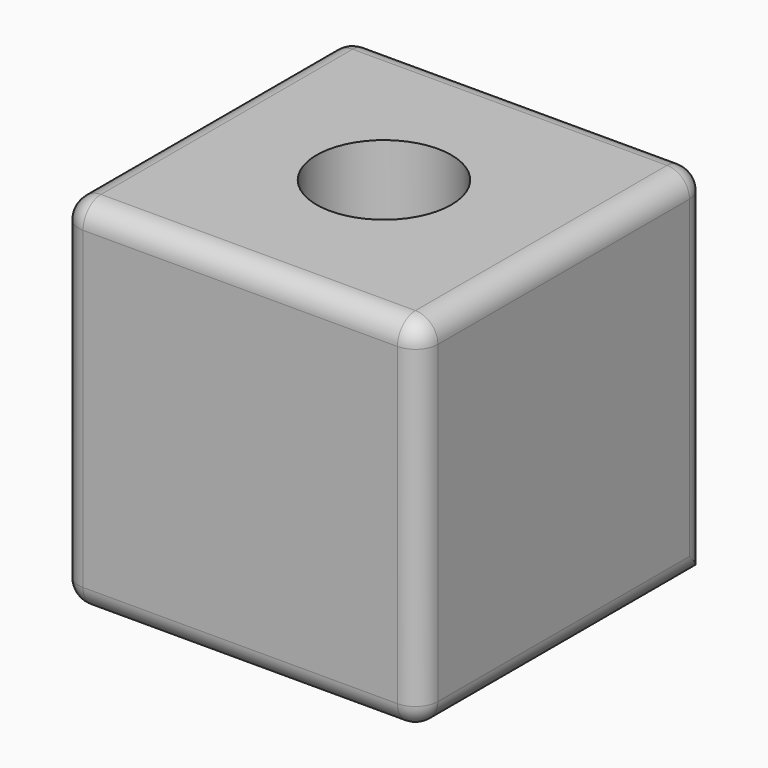
from build123d import *

# Parameters (mm, degrees)
F0_W        = 80
F0_H        = 80
F1_DEPTH    = 80
F2_R        = 5
F3_T1_DEPTH = 82.5
F3_S5_W     = 5.1
F3_S5_H     = 5.1
F3_T6_DEPTH = 5.1
F4_R        = 15
F5_DEPTH    = 80.0010001


# Not quite as in the source:
# - a fillet or chamfer that OpenCascade refuses, or shapes differently, is made with other operations: its cross-section is extruded or revolved along the edge and cut away or added


with BuildPart() as f1:
    # F0 (on Top) → F1 (new body)
    with BuildSketch(Plane.XY):
        Rectangle(F0_W, F0_H)
    extrude(amount=F1_DEPTH)

    # F2
    f2_edges = [f1.edges().sort_by_distance(p)[0] for p in [
        (0, 40, 80),
        (-40, 0, 80),
        (40, 0, 80),
        (0, -40, 80),
        (-40, 40, 40),
        (-40, 0, 0),
        (-40, -40, 40),
        (40, -40, 40),
        (0, -40, 0),
        (40, 40, 40),
        (0, 40, 0),
    ]]
    fillet(f2_edges, radius=F2_R)

    # F3: fillet of radius 5 on 8 edges, made by hand

    # F3_s2 → F3_t1 (cut)
    with BuildSketch(Plane.XZ.offset(-47.5)):
        with BuildLine():
            ThreePointArc((40, 5), (38.5355339059, 1.4644660941), (35, 0))
            Line((35, 0), (40, 0))
            Line((40, 0), (40, 5))
        make_face()
    extrude(amount=F3_T1_DEPTH, mode=Mode.SUBTRACT)


with BuildPart() as f3_tool4:
    # F3_s5 → F3_t6 (new body)
    with BuildSketch(Plane.YZ.offset(35)):
        with Locations((-37.55, 2.45)):
            Rectangle(F3_S5_W, F3_S5_H)
    extrude(amount=F3_T6_DEPTH)

    # F3_s7 → F3_t8 (revolve, cut)
    with BuildSketch(Plane(origin=(35, -35, 5), x_dir=(0, 0.7071067812, 0.7071067812), z_dir=(0, 0.7071067812, -0.7071067812))):
        with BuildLine():
            ThreePointArc((0, -5), (5, 0), (0, 5))
            Line((0, 5), (0, -5))
        make_face()
    revolve(axis=Axis((35, -35, 5), (1, 0, 0)), mode=Mode.SUBTRACT)


with BuildPart() as f1_1:
    add(f1.part)

    # F3_t3: cut F3_tool4
    add(f3_tool4.part, mode=Mode.SUBTRACT)

    # F4 (on face) → F5 (cut, through all)
    with BuildSketch(Plane.XY.offset(80)):
        Circle(F4_R)
    extrude(amount=-F5_DEPTH, mode=Mode.SUBTRACT)


solid = f1_1.part
